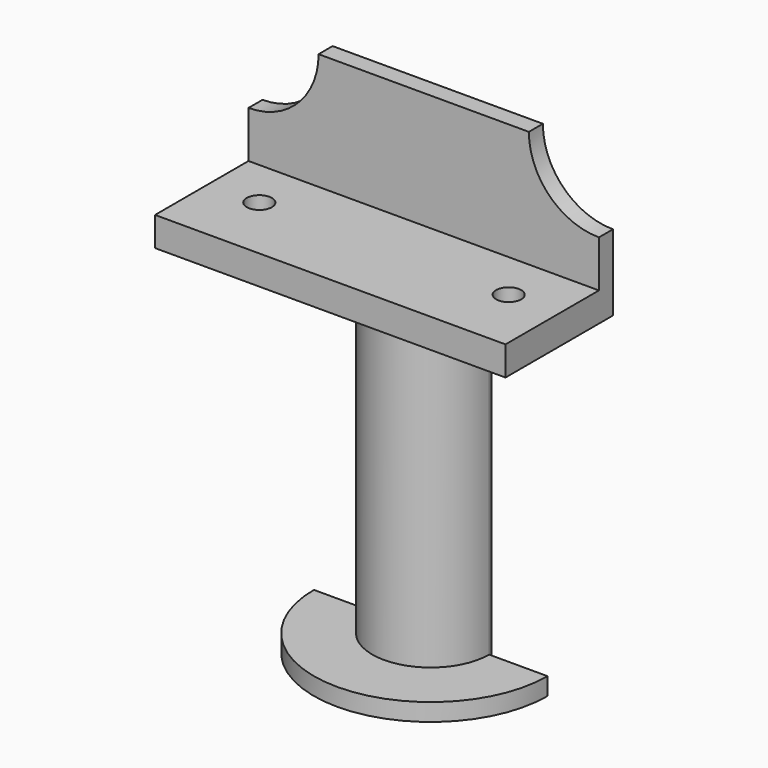
from build123d import *

# Parameters (mm, degrees)
F0_R     = 2.15
F1_DEPTH = 5
F2_W     = 60
F2_H     = 3
F3_DEPTH = 20
F5_DEPTH = 4
F6_DEPTH = 60
F8_DEPTH = 3


# Not quite as in the source:
# - a feature names something its author has since deleted; it is built from what else it names


with BuildPart() as f1:
    # F0 (on Top) → F1 (new body)
    with BuildSketch(Plane.XY):
        with BuildLine():
            ThreePointArc((-10, 4.6267989092), (-9.5606601718, 5.6874590809), (-8.5, 6.1267989092))
            Line((-8.5, 6.1267989092), (-30, 6.1267989092))
            Line((-30, 6.1267989092), (-30, -16.8732010908))
            Line((-30, -16.8732010908), (30, -16.8732010908))
            Line((30, -16.8732010908), (30, 6.1267989092))
            Line((30, 6.1267989092), (8.4999999793, 6.1267989092))
            ThreePointArc((8.4999999793, 6.1267989092), (9.5606601645, 5.6874590882), (10, 4.6267989092))
            ThreePointArc((10, 4.6267989092), (0, -5.3732010908), (-10, 4.6267989092))
        make_face()
        with Locations((-21.3480107486, -5.3732010908)):
            Circle(F0_R, mode=Mode.SUBTRACT)
        with Locations((21.3480107486, -5.3732010908)):
            Circle(F0_R, mode=Mode.SUBTRACT)
        with BuildLine():
            ThreePointArc((-7, 4.6267989092), (-7.4393398282, 5.6874590809), (-8.5, 6.1267989092))
            ThreePointArc((-8.5, 6.1267989092), (-9.5606601718, 5.6874590809), (-10, 4.6267989092))
            ThreePointArc((-10, 4.6267989092), (0, -5.3732010908), (10, 4.6267989092))
            ThreePointArc((10, 4.6267989092), (9.5606601645, 5.6874590882), (8.4999999793, 6.1267989092))
            ThreePointArc((8.4999999793, 6.1267989092), (7.4393398209, 5.6874590736), (7, 4.6267989092))
            ThreePointArc((7, 4.6267989092), (0, -2.3732010908), (-7, 4.6267989092))
        make_face()
        with BuildLine():
            Line((8, 6.1267989092), (-8, 6.1267989092))
            Line((-8, 6.1267989092), (-8.5, 6.1267989092))
            ThreePointArc((-8.5, 6.1267989092), (-7.4393398282, 5.6874590809), (-7, 4.6267989092))
            ThreePointArc((-7, 4.6267989092), (0, -2.3732010908), (7, 4.6267989092))
            ThreePointArc((7, 4.6267989092), (7.4393398209, 5.6874590736), (8.4999999793, 6.1267989092))
            Line((8.4999999793, 6.1267989092), (8, 6.1267989092))
        make_face()
    extrude(amount=F1_DEPTH)

    # F2 (on face) → F3 (join)
    with BuildSketch(Plane.XY.offset(5)):
        with Locations((0, 4.6267989092)):
            Rectangle(F2_W, F2_H)
    extrude(amount=F3_DEPTH)

    # F4 (on face) → F5 (cut)
    with BuildSketch(Plane.XZ.offset(-3.1267989092)):
        with BuildLine():
            Line((-30, 25), (-30, 13))
            ThreePointArc((-30, 13), (-21.5147186258, 16.5147186258), (-18, 25))
            Line((-18, 25), (-30, 25))
        make_face()
        with BuildLine():
            Line((30, 25), (18, 25))
            ThreePointArc((18, 25), (21.5147186258, 16.5147186258), (30, 13))
            Line((30, 13), (30, 25))
        make_face()
    extrude(amount=-F5_DEPTH, mode=Mode.SUBTRACT)

    # F0 (on Top) → F6 (join)
    with BuildSketch(Plane.XY):
        with BuildLine():
            ThreePointArc((-7, 4.6267989092), (-7.4393398282, 5.6874590809), (-8.5, 6.1267989092))
            ThreePointArc((-8.5, 6.1267989092), (-9.5606601718, 5.6874590809), (-10, 4.6267989092))
            ThreePointArc((-10, 4.6267989092), (0, -5.3732010908), (10, 4.6267989092))
            ThreePointArc((10, 4.6267989092), (9.5606601645, 5.6874590882), (8.4999999793, 6.1267989092))
            ThreePointArc((8.4999999793, 6.1267989092), (7.4393398209, 5.6874590736), (7, 4.6267989092))
            ThreePointArc((7, 4.6267989092), (0, -2.3732010908), (-7, 4.6267989092))
        make_face()
    extrude(amount=-F6_DEPTH)

    # F7 (on face) → F8 (join)
    with BuildSketch(Plane(origin=(0, 0, -60), x_dir=(1, 0, 0), z_dir=(0, 0, -1))):
        with BuildLine():
            ThreePointArc((20, -4.6267989092), (0, 15.3732010908), (-20, -4.6267989092))
            Line((-20, -4.6267989092), (-10, -4.6267989092))
            ThreePointArc((-10, -4.6267989092), (0, 5.3732010908), (10, -4.6267989092))
            Line((10, -4.6267989092), (20, -4.6267989092))
        make_face()
        with BuildLine():
            ThreePointArc((10, -4.6267989092), (0, 5.3732010908), (-10, -4.6267989092))
            Line((-10, -4.6267989092), (-7, -4.6267989092))
            ThreePointArc((-7, -4.6267989092), (0, 2.3732010908), (7, -4.6267989092))
            Line((7, -4.6267989092), (10, -4.6267989092))
        make_face()
    extrude(amount=-F8_DEPTH)


solid = f1.part
